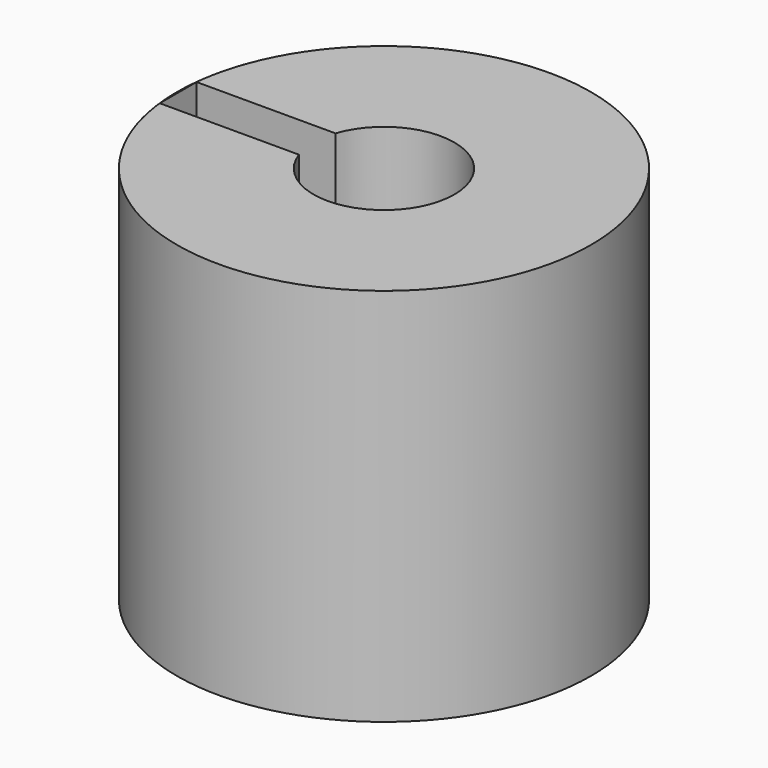
from build123d import *

# Parameters (mm, degrees)
F0_R     = 18
F1_DEPTH = 33


with BuildPart() as f1:
    # F0 (on Top) → F1 (new body)
    with BuildSketch(Plane.XY):
        Circle(F0_R)
        with BuildLine():
            ThreePointArc((-5.7976616963, 1.9755363461), (1.0012360136, 6.0426113101), (6.125, 0))
            ThreePointArc((6.125, 0), (1.0012360136, -6.0426113101), (-5.7976616963, -1.9755363461))
            Line((-5.7976616963, -1.9755363461), (-5.7976616963, -2.0244636539))
            Line((-5.7976616963, -2.0244636539), (-17.8778566858, -2.0244636539))
            Line((-17.8778566858, -2.0244636539), (-17.8778566858, 1.9755363461))
            Line((-17.8778566858, 1.9755363461), (-5.7976616963, 1.9755363461))
        make_face(mode=Mode.SUBTRACT)
    extrude(amount=F1_DEPTH)


solid = f1.part
